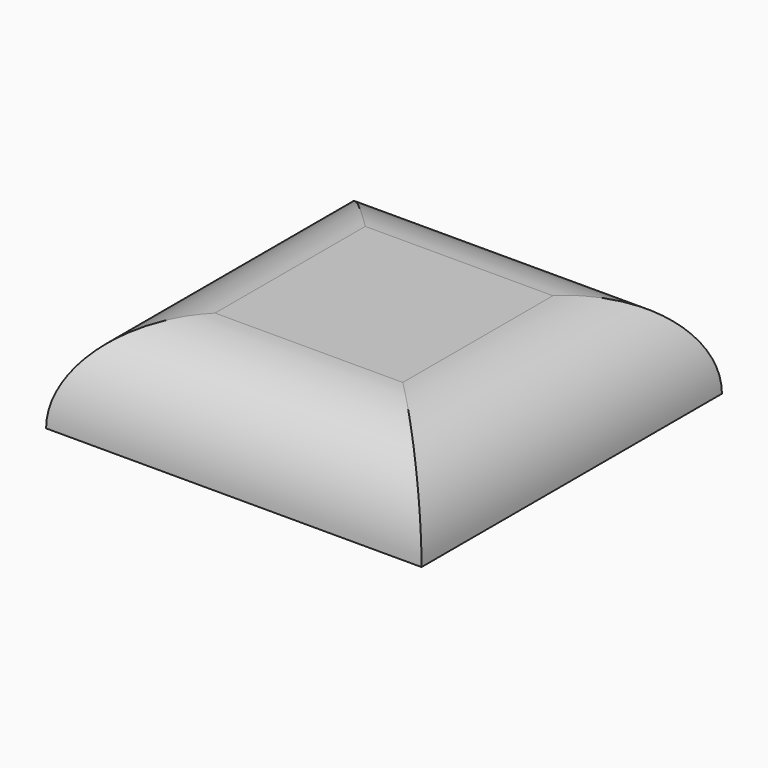
from build123d import *

# Parameters (mm, degrees)
F3_W     = 50.7285948843
F3_H     = 69.9163675308
F6_W     = 101.6
F6_H     = 101.6
F7_DEPTH = 25.4
F8_R     = 25.39999


# Not quite as in the source:
# - a fillet or chamfer is up to 0.001 mm smaller than in the source, because OpenCascade refuses the exact size


with BuildPart() as f4:
    # F1 (on offset) → F4 section 0
    with BuildSketch(Plane.YZ.offset(127)):
        with BuildLine():
            add(Edge.make_bspline(
                [(-11.8536790833, -25.3428127617), (16.5973998136, -117.2622232897), (89.6947664905, -44.2741583201), (162.7921331674, 28.7139066495), (61.2436875936, 47.6452522079), (-40.3047579802, 66.5765977664), (-11.8536790833, -25.3428127617)],
                knots=[0, 0, 0, 2.0943951024, 2.0943951024, 4.1887902048, 4.1887902048, 6.2831853072, 6.2831853072, 6.2831853072], degree=2, weights=[1, 0.5, 1, 0.5, 1, 0.5, 1]))
        make_face()
    # F3 (on offset) → F4 section 1
    with BuildSketch(Plane.XY.offset(254)):
        with Locations((-8.5154855624, -1.6246475279)):
            Rectangle(F3_W, F3_H)
    loft()


with BuildPart() as f7:
    # F6 (on offset) → F7 (new body)
    with BuildSketch(Plane.XY.offset(254)):
        with Locations((-0.4687514156, 6.5054772415)):
            Rectangle(F6_W, F6_H)
    extrude(amount=F7_DEPTH)

    # F8 (radius 25.4 in the source; OpenCascade refuses exactly that, so slightly less here)
    f8_edges = [f7.edges().sort_by_distance(p)[0] for p in [
        (50.331249, 6.505477, 279.4),
        (-0.468751, 57.305477, 279.4),
        (-51.268751, 6.505477, 279.4),
        (-0.468751, -44.294523, 279.4),
    ]]
    fillet(f8_edges, radius=F8_R)


solid = f7.part
